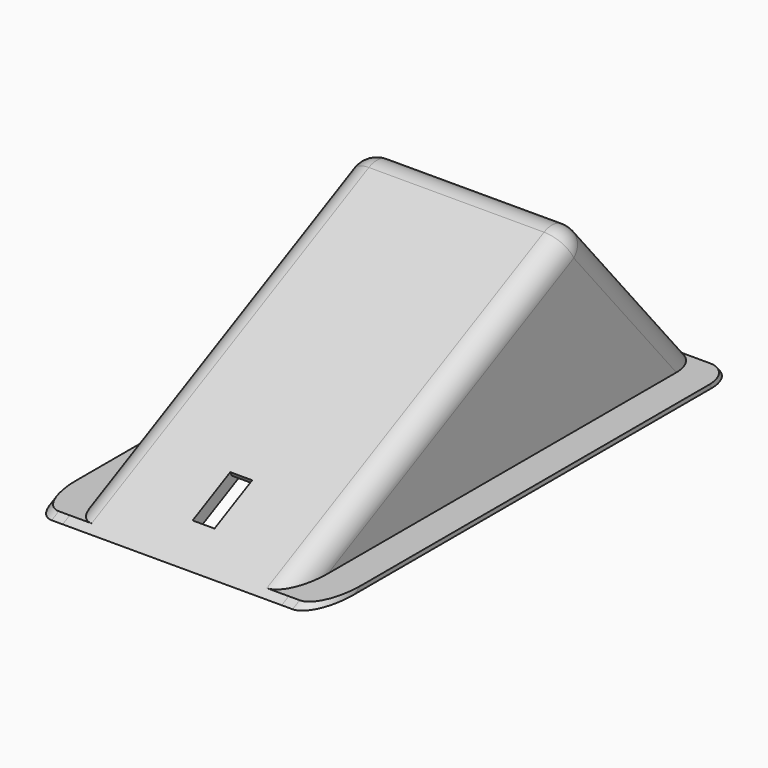
from build123d import *

# Parameters (mm, degrees)
F1_DEPTH      = 50
F2_DEPTH      = 3
F4_DEPTH      = 3
F5_W          = 30
F5_H          = 2
F6_DEPTH      = 25
F7_W          = 5
F7_H          = 12
F8_DEPTH      = 25
F9_SIZE       = 2
F11_DEPTH     = 7.5
F12_T1_DEPTH  = 26.3054072893
F13_T1_DEPTH  = 27.2441766919
F15_DEPTH     = 7.5
F16_T1_DEPTH  = 26.3054072893
F17_T1_DEPTH  = 27.2441766919
F18_R         = 5
F19_T4_DEPTH  = 100.8695078042
F19_T7_ANGLE  = 76.4615865705
F19_T11_DEPTH = 62.2556275763
F20_T4_DEPTH  = 100.8695078042
F20_T9_DEPTH  = 62.2556275763
F20_T12_ANGLE = 76.4615865705


# Not quite as in the source:
# - a fillet or chamfer that OpenCascade refuses, or shapes differently, is made with other operations: its cross-section is extruded or revolved along the edge and cut away or added


with BuildPart() as f1:
    # F0 (on Right) → F1 (new body)
    with BuildSketch(Plane.YZ):
        Polygon((28.4014230277, 3.870410641), (-56.2452584396, -38.2620337305), (-49.5127283639, -38.2620337305), (27.6224404883, 0.1315944002), (59.8385196924, -38.2620337305), (63.7547415604, -38.2620337305), align=None)
    extrude(amount=F1_DEPTH)

    # F0 (on Right) → F2 (join)
    with BuildSketch(Plane.YZ):
        Polygon((27.6224404883, 0.1315944002), (-49.5127283639, -38.2620337305), (59.8385196924, -38.2620337305), align=None)
    extrude(amount=F2_DEPTH)

    # F3 (on face) → F4 (join)
    with BuildSketch(Plane.YZ.offset(50)):
        Polygon((27.6224404883, 0.1315944002), (-49.5127283639, -38.2620337305), (59.8385196924, -38.2620337305), align=None)
    extrude(amount=-F4_DEPTH)

    # F5 (on face) → F6 (cut)
    with BuildSketch(Plane(origin=(0, 18.5724443931, 15.5841312403), x_dir=(-1, 0, 0), z_dir=(0, 0.7660444431, 0.6427876097))):
        with Locations((-25, -42.7911762555)):
            Rectangle(F5_W, F5_H)
    extrude(amount=-F6_DEPTH, mode=Mode.SUBTRACT)

    # F7 (on face) → F8 (cut)
    with BuildSketch(Plane(origin=(0, 4.0953498153, -8.2278105741), x_dir=(1, 0, 0), z_dir=(0, -0.4455977123, 0.8952333097))):
        with Locations((25, -51.4021035664)):
            Rectangle(F7_W, F7_H)
    extrude(amount=-F8_DEPTH, mode=Mode.SUBTRACT)

    # F9
    f9_edges = [f1.edges().sort_by_distance(p)[0] for p in [
        (25, -35.213332, -31.144584),
    ]]
    chamfer(f9_edges, length=F9_SIZE)

    # F10 (on face) → F11 (join)
    with BuildSketch(Plane(origin=(0, 0, 0), x_dir=(0, -1, 0), z_dir=(-1, 0, 0))):
        Polygon((56.2452584396, -38.2620337305), (54.2361967122, -37.2620337305), (-62.9156419292, -37.2620337305), (-63.7547415604, -38.2620337305), align=None)
    extrude(amount=F11_DEPTH)

    # F12: fillet of radius 5 on 1 edges, made by hand

    # F12_s2 → F12_t1 (cut)
    with BuildSketch(Plane(origin=(0, 36.3083524151, -43.2706094318), x_dir=(1, 0, 0), z_dir=(0, 0.6427876097, -0.7660444431))):
        with BuildLine():
            ThreePointArc((-7.5, -19.2446042914), (-6.0355339059, -22.7801381974), (-2.5, -24.2446042914))
            Line((-2.5, -24.2446042914), (-7.5, -24.2446042914))
            Line((-7.5, -24.2446042914), (-7.5, -19.2446042914))
        make_face()
    extrude(amount=F12_T1_DEPTH, mode=Mode.SUBTRACT)

    # F13: fillet of radius 5 on 1 edges, made by hand

    # F13_s2 → F13_t1 (cut)
    with BuildSketch(Plane(origin=(0, -71.5310246258, -35.6041945608), x_dir=(1, 0, 0), z_dir=(0, 0.8952333097, 0.4455977123))):
        with BuildLine():
            ThreePointArc((-2.5, 9.1906886005), (-6.0355339059, 10.6551546946), (-7.5, 14.1906886005))
            Line((-7.5, 14.1906886005), (-7.5, 9.1906886005))
            Line((-7.5, 9.1906886005), (-2.5, 9.1906886005))
        make_face()
    extrude(amount=F13_T1_DEPTH, mode=Mode.SUBTRACT)

    # F14 (on face) → F15 (join)
    with BuildSketch(Plane.YZ.offset(50)):
        Polygon((63.7547415604, -38.2620337305), (62.9156419292, -37.2620337305), (-54.2361967122, -37.2620337305), (-56.2452584396, -38.2620337305), align=None)
    extrude(amount=F15_DEPTH)

    # F16: fillet of radius 5 on 1 edges, made by hand

    # F16_s2 → F16_t1 (cut)
    with BuildSketch(Plane(origin=(0, 53.2171422884, -63.4217205098), x_dir=(1, 0, 0), z_dir=(0, -0.6427876097, 0.7660444431))):
        with BuildLine():
            ThreePointArc((52.5, 24.2446042914), (56.0355339059, 22.7801381974), (57.5, 19.2446042914))
            Line((57.5, 19.2446042914), (57.5, 24.2446042914))
            Line((57.5, 24.2446042914), (52.5, 24.2446042914))
        make_face()
    extrude(amount=F16_T1_DEPTH, mode=Mode.SUBTRACT)

    # F17: fillet of radius 5 on 1 edges, made by hand

    # F17_s2 → F17_t1 (cut)
    with BuildSketch(Plane(origin=(0, -47.1411301566, -23.4642517522), x_dir=(1, 0, 0), z_dir=(0, -0.8952333097, -0.4455977123))):
        with BuildLine():
            ThreePointArc((52.5, -9.1906886005), (56.0355339059, -10.6551546946), (57.5, -14.1906886005))
            Line((57.5, -14.1906886005), (57.5, -9.1906886005))
            Line((57.5, -9.1906886005), (52.5, -9.1906886005))
        make_face()
    extrude(amount=F17_T1_DEPTH, mode=Mode.SUBTRACT)

    # F18
    f18_edges = [f1.edges().sort_by_distance(p)[0] for p in [
        (25, 28.401423, 3.870411),
    ]]
    fillet(f18_edges, radius=F18_R)

    # F19: fillet of radius 5 on 3 edges, made by hand


with BuildPart() as f19_tool2:
    # F19_s3 → F19_t4 (new body)
    with BuildSketch(Plane(origin=(0, 20.7797804184, 10.3430273622), x_dir=(1, 0, 0), z_dir=(0, -0.8952333097, -0.4455977123))):
        with BuildLine():
            ThreePointArc((45, -9.1906886005), (48.5355339059, -10.6551546946), (50, -14.1906886005))
            Line((50, -14.1906886005), (50, -9.1906886005))
            Line((50, -9.1906886005), (45, -9.1906886005))
        make_face()
    extrude(amount=F19_T4_DEPTH)

    split(bisect_by=Plane.XY.offset(-37.2620337305), keep=Keep.TOP)


with BuildPart() as f1_1:
    add(f1.part)

    # F19_t1: cut F19_tool2
    add(f19_tool2.part, mode=Mode.SUBTRACT)

    # F19_s6 → F19_t7 (revolve, cut)
    with BuildSketch(Plane(origin=(0, 20.7797804184, 10.3430273622), x_dir=(1, 0, 0), z_dir=(0, -0.8952333097, -0.4455977123))):
        with BuildLine():
            ThreePointArc((45, -9.1906886005), (48.5355339059, -10.6551546946), (50, -14.1906886005))
            Line((50, -14.1906886005), (50, -9.1906886005))
            Line((50, -9.1906886005), (45, -9.1906886005))
        make_face()
    revolve(axis=Axis((50, 27.1031187954, -2.3609497603), (-1, 0, 0)), revolution_arc=F19_T7_ANGLE, mode=Mode.SUBTRACT)


with BuildPart() as f19_tool9:
    # F19_s10 → F19_t11 (new body)
    with BuildSketch(Plane(origin=(0, 52.3780426572, -62.4217205098), x_dir=(1, 0, 0), z_dir=(0, -0.6427876097, 0.7660444431))):
        with BuildLine():
            ThreePointArc((50, 19.2446042914), (48.5355339059, 22.7801381974), (45, 24.2446042914))
            Line((45, 24.2446042914), (50, 24.2446042914))
            Line((50, 24.2446042914), (50, 19.2446042914))
        make_face()
    extrude(amount=F19_T11_DEPTH)

    split(bisect_by=Plane.XY.offset(-37.2620337305), keep=Keep.TOP)


with BuildPart() as f1_2:
    add(f1_1.part)

    # F19_t8: cut F19_tool9
    add(f19_tool9.part, mode=Mode.SUBTRACT)

    # F20: fillet of radius 5 on 3 edges, made by hand


with BuildPart() as f20_tool2:
    # F20_s3 → F20_t4 (new body)
    with BuildSketch(Plane(origin=(0, 20.7797804184, 10.3430273622), x_dir=(1, 0, 0), z_dir=(0, -0.8952333097, -0.4455977123))):
        with BuildLine():
            ThreePointArc((5, -9.1906886005), (1.4644660941, -10.6551546946), (0, -14.1906886005))
            Line((0, -14.1906886005), (0, -9.1906886005))
            Line((0, -9.1906886005), (5, -9.1906886005))
        make_face()
    extrude(amount=F20_T4_DEPTH)

    split(bisect_by=Plane.XY.offset(-37.2620337305), keep=Keep.TOP)


with BuildPart() as f1_3:
    add(f1_2.part)

    # F20_t1: cut F20_tool2
    add(f20_tool2.part, mode=Mode.SUBTRACT)


with BuildPart() as f20_tool7:
    # F20_s8 → F20_t9 (new body)
    with BuildSketch(Plane(origin=(0, 52.3780426572, -62.4217205098), x_dir=(1, 0, 0), z_dir=(0, -0.6427876097, 0.7660444431))):
        with BuildLine():
            ThreePointArc((0, 19.2446042914), (1.4644660941, 22.7801381974), (5, 24.2446042914))
            Line((5, 24.2446042914), (0, 24.2446042914))
            Line((0, 24.2446042914), (0, 19.2446042914))
        make_face()
    extrude(amount=F20_T9_DEPTH)

    split(bisect_by=Plane.XY.offset(-37.2620337305), keep=Keep.TOP)


with BuildPart() as f1_4:
    add(f1_3.part)

    # F20_t6: cut F20_tool7
    add(f20_tool7.part, mode=Mode.SUBTRACT)

    # F20_s11 → F20_t12 (revolve, cut)
    with BuildSketch(Plane(origin=(0, 20.7797804184, 10.3430273622), x_dir=(1, 0, 0), z_dir=(0, -0.8952333097, -0.4455977123))):
        with BuildLine():
            ThreePointArc((0, -14.1906886005), (1.4644660941, -10.6551546946), (5, -9.1906886005))
            Line((5, -9.1906886005), (0, -9.1906886005))
            Line((0, -9.1906886005), (0, -14.1906886005))
        make_face()
    revolve(axis=Axis((0, 27.1031187954, -2.3609497603), (-1, 0, 0)), revolution_arc=F20_T12_ANGLE, mode=Mode.SUBTRACT)


solid = f1_4.part
